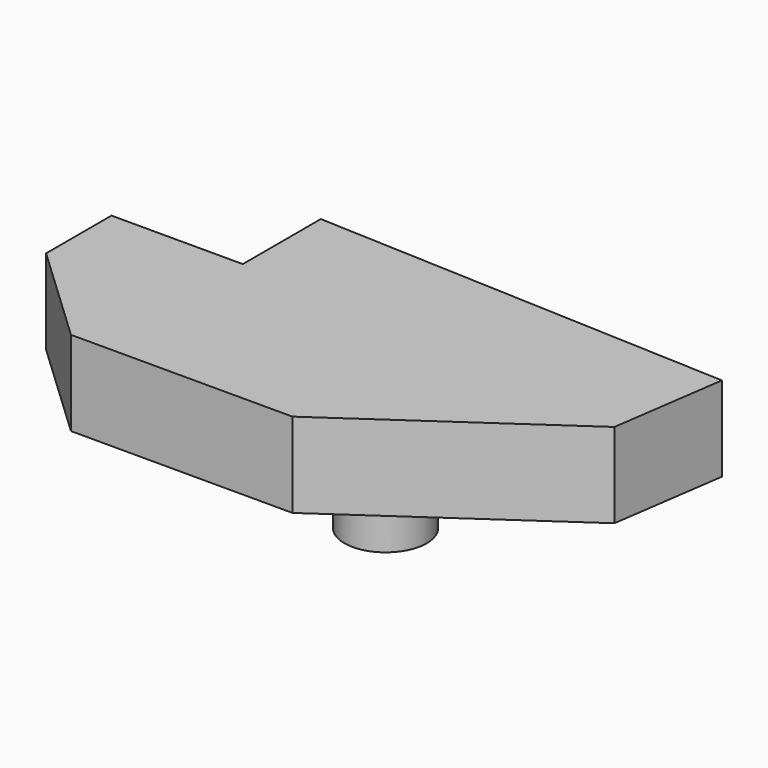
from build123d import *

# Parameters (mm, degrees)
F1_DEPTH = 33.3509109914
F2_R     = 16.1774889393
F3_DEPTH = 39.8117862642


# Not quite as in the source:
# - a feature names something its author has since deleted; it is built from what else it names


with BuildPart() as f1:
    # F0 (on Top) → F1 (new body)
    with BuildSketch(Plane.XY):
        Polygon((75.3069221973, -69.7055906057), (156.8375527859, -13.2772475481), (160.0531488657, 9.1281235218), (163.2687449455, 31.5334945917), (0, 38.3795797825), (0, 0), (-51.6568571329, 0), (-51.6568571329, -32.155841589), (-11.8250846863, -69.7055906057), align=None)
    extrude(amount=F1_DEPTH)

    # F2 (on Top) → F3 (join)
    with BuildSketch(Plane.XY):
        with Locations((56.1946332455, 0)):
            Circle(F2_R)
    extrude(amount=-F3_DEPTH)


solid = f1.part
